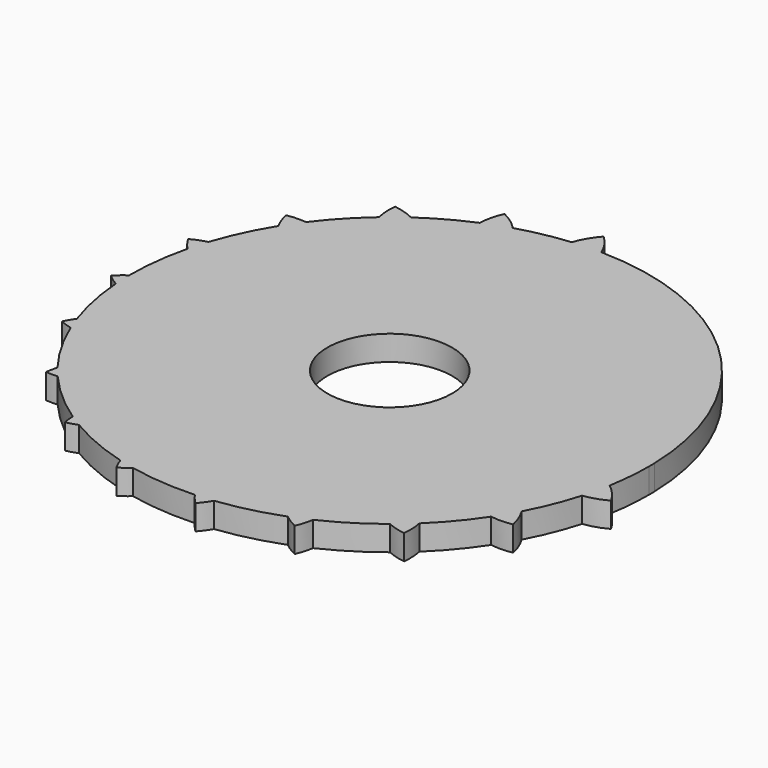
from build123d import *

# Parameters (mm, degrees)
F1_R     = 2.5
F2_DEPTH = 1


with BuildPart() as f2:
    # F1 (on Top) → F2 (new body)
    with BuildSketch(Plane.XY):
        with BuildLine():
            ThreePointArc((10.4010177666, 0.2791052033), (7.3183650566, 7.3959856133), (0.1693586543, 10.4033834852))
            ThreePointArc((0.1693586543, 10.4033834852), (-0.4084890354, 10.3967402104), (-0.9850766389, 10.358025599))
            ThreePointArc((-0.9850766389, 10.358025599), (-2.0168567686, 10.2074168657), (-3.0283814682, 9.9542943486))
            ThreePointArc((-3.0283814682, 9.9542943486), (-3.5459501656, 9.7818867156), (-4.0537711259, 9.5825888962))
            ThreePointArc((-4.0537711259, 9.5825888962), (-5.0373972408, 9.1040485134), (-5.9653480877, 8.5248866554))
            ThreePointArc((-5.9653480877, 8.5248866554), (-6.3706851973, 8.2263868382), (-6.7611105438, 7.9086316458))
            ThreePointArc((-6.7611105438, 7.9086316458), (-7.5960763624, 7.1104637114), (-8.3374242637, 6.2246627975))
            ThreePointArc((-8.3374242637, 6.2246627975), (-8.6009812596, 5.8550996291), (-8.8481688232, 5.4743930047))
            ThreePointArc((-8.8481688232, 5.4743930047), (-9.4287165512, 4.3998152793), (-9.8793415326, 3.2646104174))
            ThreePointArc((-9.8793415326, 3.2646104174), (-9.9979773753, 2.8808885258), (-10.1017152215, 2.4928738192))
            ThreePointArc((-10.1017152215, 2.4928738192), (-10.3320366233, 1.228042959), (-10.4046136849, -0.0555370437))
            ThreePointArc((-10.4046136849, -0.0555370437), (-10.3967402104, -0.4084890354), (-10.3768971195, -0.7609707396))
            ThreePointArc((-10.3768971195, -0.7609707396), (-10.193126284, -2.0878809482), (-9.8403979466, -3.3801832122))
            ThreePointArc((-9.8403979466, -3.3801832122), (-9.7333865621, -3.676990118), (-9.6174251884, -3.9704159783))
            ThreePointArc((-9.6174251884, -3.9704159783), (-9.0097773066, -5.204131357), (-8.2447283135, -6.3469303865))
            ThreePointArc((-8.2447283135, -6.3469303865), (-8.061087037, -6.5785975768), (-7.8709383234, -6.8049540927))
            ThreePointArc((-7.8709383234, -6.8049540927), (-6.8959867768, -7.7913051967), (-5.7985154997, -8.6392296123))
            ThreePointArc((-5.7985154997, -8.6392296123), (-5.549424479, -8.8013043491), (-5.2958064015, -8.9561992414))
            ThreePointArc((-5.2958064015, -8.9561992414), (-4.0708941637, -9.5753272008), (-2.7751475554, -10.0278425566))
            ThreePointArc((-2.7751475554, -10.0278425566), (-2.4655602512, -10.1084164409), (-2.1536422724, -10.1794349184))
            ThreePointArc((-2.1536422724, -10.1794349184), (-0.8330496502, -10.3713595336), (0.5012461634, -10.3926812026))
            ThreePointArc((0.5012461634, -10.3926812026), (0.8600204589, -10.3691578783), (1.2177678025, -10.3332527248))
            ThreePointArc((1.2177678025, -10.3332527248), (2.476254211, -10.105802065), (3.6973306562, -9.725678193))
            ThreePointArc((3.6973306562, -9.725678193), (4.0769602691, -9.5727459623), (4.4502816898, -9.4050020296))
            ThreePointArc((4.4502816898, -9.4050020296), (5.5153513374, -8.8226962954), (6.5053546396, -8.1203098037))
            ThreePointArc((6.5053546396, -8.1203098037), (6.8591715093, -7.823735457), (7.1994838987, -7.5117575764))
            ThreePointArc((7.1994838987, -7.5117575764), (7.983010793, -6.6731258772), (8.6694062261, -5.7533004425))
            ThreePointArc((8.6694062261, -5.7533004425), (8.9411374277, -5.3211964626), (9.1913496147, -4.8762857335))
            ThreePointArc((9.1913496147, -4.8762857335), (9.6500459533, -3.8904605631), (10.0033580362, -2.8621492438))
            ThreePointArc((10.0033580362, -2.8621492438), (10.1409184183, -2.3282705875), (10.2500070535, -1.7878550549))
            ThreePointArc((10.2500070535, -1.7878550549), (10.3660009938, -0.8972701323), (10.4047619048, 0))
            ThreePointArc((10.4047619048, 0), (10.4038258281, 0.1395651578), (10.4010177666, 0.2791052033))
        make_face()
        Circle(F1_R, mode=Mode.SUBTRACT)
        with BuildLine():
            ThreePointArc((-0.9850766389, 10.358025599), (-0.4084890354, 10.3967402104), (0.1693586543, 10.4033834852))
            ThreePointArc((0.1693586543, 10.4033834852), (-0.0915577789, 10.8736948256), (-0.4432176074, 11.280641391))
            ThreePointArc((-0.4432176074, 11.280641391), (-0.7618647264, 10.8473583939), (-0.9850766389, 10.358025599))
        make_face()
        with BuildLine():
            ThreePointArc((-4.0537711259, 9.5825888962), (-3.5459501656, 9.7818867156), (-3.0283814682, 9.9542943486))
            ThreePointArc((-3.0283814682, 9.9542943486), (-3.3994309889, 10.2837794802), (-3.8260663696, 10.5371970223))
            ThreePointArc((-3.8260663696, 10.5371970223), (-3.9851262119, 10.0706763942), (-4.0537711259, 9.5825888962))
        make_face()
        with BuildLine():
            ThreePointArc((10.9249748031, -2.5617942214), (10.6258758179, -2.1413484121), (10.2500070535, -1.7878550549))
            ThreePointArc((10.2500070535, -1.7878550549), (10.1409184183, -2.3282705875), (10.0033580362, -2.8621492438))
            ThreePointArc((10.0033580362, -2.8621492438), (10.4782123863, -2.7550707236), (10.9249748031, -2.5617942214))
        make_face()
        with BuildLine():
            ThreePointArc((-6.7611105438, 7.9086316458), (-6.3706851973, 8.2263868382), (-5.9653480877, 8.5248866554))
            ThreePointArc((-5.9653480877, 8.5248866554), (-6.3783708882, 8.691089302), (-6.8136097843, 8.784781654))
            ThreePointArc((-6.8136097843, 8.784781654), (-6.8244021361, 8.3444870809), (-6.7611105438, 7.9086316458))
        make_face()
        with BuildLine():
            ThreePointArc((9.5380453186, -5.7355619953), (9.4030800104, -5.2904375026), (9.1913496147, -4.8762857335))
            ThreePointArc((9.1913496147, -4.8762857335), (8.9411374277, -5.3211964626), (8.6694062261, -5.7533004425))
            ThreePointArc((8.6694062261, -5.7533004425), (9.1044680071, -5.7807779267), (9.5380453186, -5.7355619953))
        make_face()
        with BuildLine():
            ThreePointArc((-8.8481688232, 5.4743930047), (-8.6009812596, 5.8550996291), (-8.3374242637, 6.2246627975))
            ThreePointArc((-8.3374242637, 6.2246627975), (-8.7265255483, 6.2387786553), (-9.1134062865, 6.1949339122))
            ThreePointArc((-9.1134062865, 6.1949339122), (-9.0073910178, 5.8248704891), (-8.8481688232, 5.4743930047))
        make_face()
        with BuildLine():
            ThreePointArc((7.2382488163, -8.3254097371), (7.2507593771, -7.9170641742), (7.1994838987, -7.5117575764))
            ThreePointArc((7.1994838987, -7.5117575764), (6.8591715093, -7.823735457), (6.5053546396, -8.1203098037))
            ThreePointArc((6.5053546396, -8.1203098037), (6.8642964884, -8.2496786303), (7.2382488163, -8.3254097371))
        make_face()
        with BuildLine():
            ThreePointArc((-10.1017152215, 2.4928738192), (-9.9979773753, 2.8808885258), (-9.8793415326, 3.2646104174))
            ThreePointArc((-9.8793415326, 3.2646104174), (-10.1976364828, 3.162779516), (-10.500335771, 3.0211661383))
            ThreePointArc((-10.500335771, 3.0211661383), (-10.3178144144, 2.7443519774), (-10.1017152215, 2.4928738192))
        make_face()
        with BuildLine():
            ThreePointArc((4.2507054017, -10.0778251054), (4.373179067, -9.7481426651), (4.4502816898, -9.4050020296))
            ThreePointArc((4.4502816898, -9.4050020296), (4.0769602691, -9.5727459623), (3.6973306562, -9.725678193))
            ThreePointArc((3.6973306562, -9.725678193), (3.9629273196, -9.919179939), (4.2507054017, -10.0778251054))
        make_face()
        with BuildLine():
            ThreePointArc((-10.3768971195, -0.7609707396), (-10.3967402104, -0.4084890354), (-10.4046136849, -0.0555370437))
            ThreePointArc((-10.4046136849, -0.0555370437), (-10.6317595983, -0.2288157362), (-10.8386359166, -0.425851165))
            ThreePointArc((-10.8386359166, -0.425851165), (-10.6169381073, -0.6060478704), (-10.3768971195, -0.7609707396))
        make_face()
        with BuildLine():
            ThreePointArc((0.8678566395, -10.8212694742), (1.0568743578, -10.5873437424), (1.2177678025, -10.3332527248))
            ThreePointArc((1.2177678025, -10.3332527248), (0.8600204589, -10.3691578783), (0.5012461634, -10.3926812026))
            ThreePointArc((0.5012461634, -10.3926812026), (0.6729569444, -10.6168931305), (0.8678566395, -10.8212694742))
        make_face()
        with BuildLine():
            ThreePointArc((-9.6174251884, -3.9704159783), (-9.7333865621, -3.676990118), (-9.8403979466, -3.3801832122))
            ThreePointArc((-9.8403979466, -3.3801832122), (-9.978035392, -3.5883525406), (-10.0951915478, -3.8086999272))
            ThreePointArc((-10.0951915478, -3.8086999272), (-9.8602185944, -3.901110143), (-9.6174251884, -3.9704159783))
        make_face()
        with BuildLine():
            ThreePointArc((-2.5791606638, -10.4829693286), (-2.3587946678, -10.341865934), (-2.1536422724, -10.1794349184))
            ThreePointArc((-2.1536422724, -10.1794349184), (-2.4655602512, -10.1084164409), (-2.7751475554, -10.0278425566))
            ThreePointArc((-2.7751475554, -10.0278425566), (-2.6879646474, -10.2600611812), (-2.5791606638, -10.4829693286))
        make_face()
        with BuildLine():
            ThreePointArc((-7.8709383234, -6.8049540927), (-8.061087037, -6.5785975768), (-8.2447283135, -6.3469303865))
            ThreePointArc((-8.2447283135, -6.3469303865), (-8.3036538881, -6.5694261546), (-8.3427761795, -6.7962433419))
            ThreePointArc((-8.3427761795, -6.7962433419), (-8.1070542554, -6.8112698876), (-7.8709383234, -6.8049540927))
        make_face()
        with BuildLine():
            ThreePointArc((-5.7529284377, -9.0960398441), (-5.5211636058, -9.036592423), (-5.2958064015, -8.9561992414))
            ThreePointArc((-5.2958064015, -8.9561992414), (-5.549424479, -8.8013043491), (-5.7985154997, -8.6392296123))
            ThreePointArc((-5.7985154997, -8.6392296123), (-5.7857710928, -8.8686375736), (-5.7529284377, -9.0960398441))
        make_face()
    extrude(amount=F2_DEPTH)


solid = f2.part
